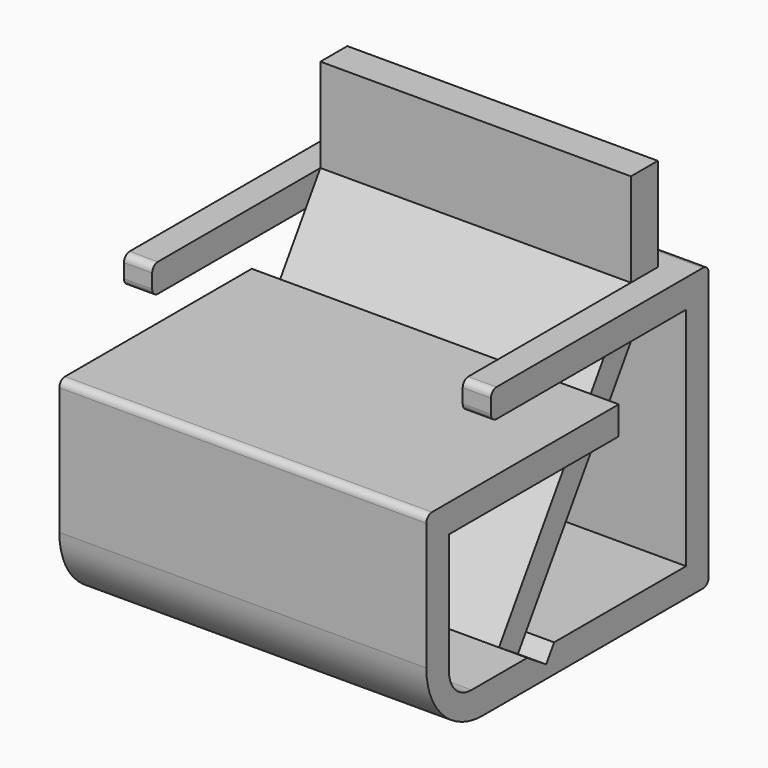
from build123d import *

# Parameters (mm, degrees)
F1_DEPTH = 660.4
F3_DEPTH = 86.54255
F5_DEPTH = 558.8
F7_DEPTH = 762
F8_R     = 12.7


# Not quite as in the source:
# - a feature of the source that left no trace in its solid (it failed there, or was rolled back) is left out


with BuildPart() as f1:
    # F0 (on Right) → F1 (new body)
    with BuildSketch(Plane.YZ):
        with BuildLine():
            Line((324.2077479366, 0), (324.2077479366, 508))
            Line((324.2077479366, 508), (-165.4576212168, 508))
            Line((-165.4576212168, 508), (-165.4576212168, 457.2))
            Line((-165.4576212168, 457.2), (273.4077479366, 457.2))
            Line((273.4077479366, 457.2), (273.4077479366, 50.8))
            Line((273.4077479366, 50.8), (-209.1922520634, 50.8))
            ThreePointArc((-209.1922520634, 50.8), (-245.1132765477, 65.6789755157), (-259.9922520634, 101.6))
            Line((-259.9922520634, 101.6), (-259.9922520634, 317.9801367223))
            Line((-259.9922520634, 317.9801367223), (121.9838493824, 317.9801367223))
            Line((121.9838493824, 317.9801367223), (121.9838493824, 368.7801367223))
            Line((121.9838493824, 368.7801367223), (-310.7922520634, 368.7801367223))
            Line((-310.7922520634, 368.7801367223), (-310.7922520634, 127))
            ThreePointArc((-310.7922520634, 127), (-273.5948132741, 37.1974387893), (-183.7922520634, 0))
            Line((-183.7922520634, 0), (324.2077479366, 0))
        make_face()
    extrude(amount=F1_DEPTH)

    # F2 (on face) → F3 (cut)
    with BuildSketch(Plane.XY.offset(508)):
        Polygon((50.8, 273.4077479366), (50.8, -114.6576212168), (50.8, -165.4576212168), (609.6, -165.4576212168), (609.6, -114.6576212168), (609.6, 273.4077479366), align=None)
    extrude(amount=-F3_DEPTH, mode=Mode.SUBTRACT)

    # F6 (on face) → F7 (cut)
    with BuildSketch(Plane(origin=(0, 0, 0), x_dir=(0, -1, 0), z_dir=(-1, 0, 0))):
        Polygon((23.3521865532, 50.8), (41.3043974346, 23.1421194673), (83.9152134845, 50.8), align=None)
    extrude(amount=-F7_DEPTH, mode=Mode.SUBTRACT)

    # F8
    f8_edges = [f1.edges().sort_by_distance(p)[0] for p in [
        (330.2, 324.207748, 0),
        (330.2, 324.207748, 508),
        (25.4, -165.457621, 508),
        (25.4, -165.457621, 457.2),
        (635, -165.457621, 508),
        (635, -165.457621, 457.2),
        (330.2, -310.792252, 368.780137),
    ]]
    fillet(f8_edges, radius=F8_R)


with BuildPart() as f5:
    # F4 (on face) → F5 (new body, through all)
    with BuildSketch(Plane(origin=(609.6, 0, 0), x_dir=(0, -1, 0), z_dir=(-1, 0, 0))):
        Polygon((-273.4077479366, 676.4837503433), (-273.4077479366, 508), (41.3043974346, 23.1421194673), (83.9152134845, 50.8), (-212.8447210052, 508), (-212.8447210052, 676.4837503433), align=None)
    extrude(amount=F5_DEPTH)


solid = Compound([f1.part, f5.part])
